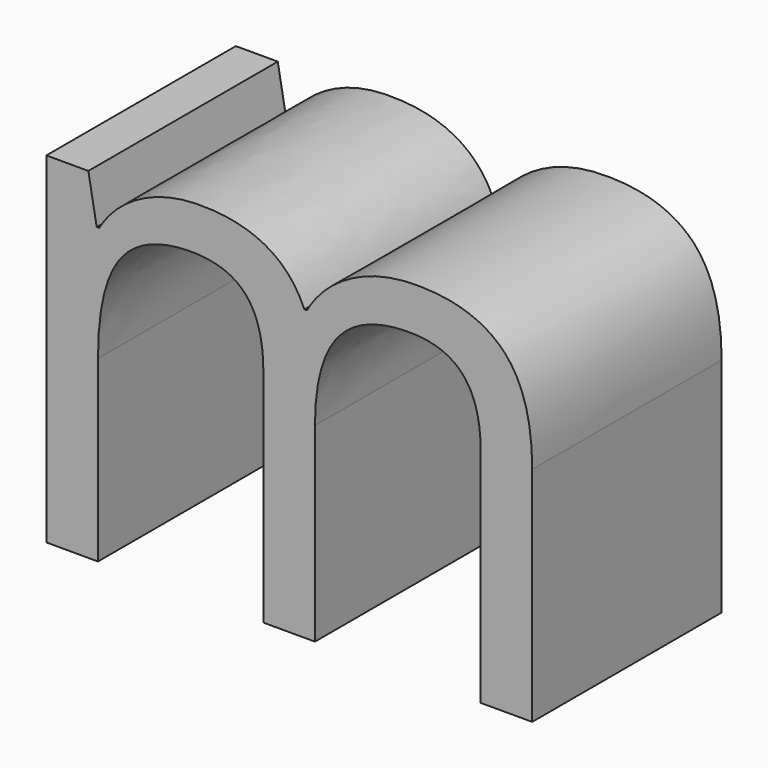
from build123d import *

# Parameters (mm, degrees)
F0_TEXT_SIZE = 34.149728405
F1_DEPTH     = 12.7


# Not quite as in the source:
# - Text() gives the source's letters only with a copy of the font that has no kerning and outlines rounded to 1/6400 em; it was checked with that copy


with BuildPart() as f1:
    # F0 (on Front) → F1 (new body)
    with BuildSketch(Plane.XZ):
        with Locations((-58.9707568288, 0)):
            Text('m', F0_TEXT_SIZE, font='Open Sans', text_align=(TextAlign.LEFT, TextAlign.BOTTOM))
    extrude(amount=F1_DEPTH)


solid = f1.part
